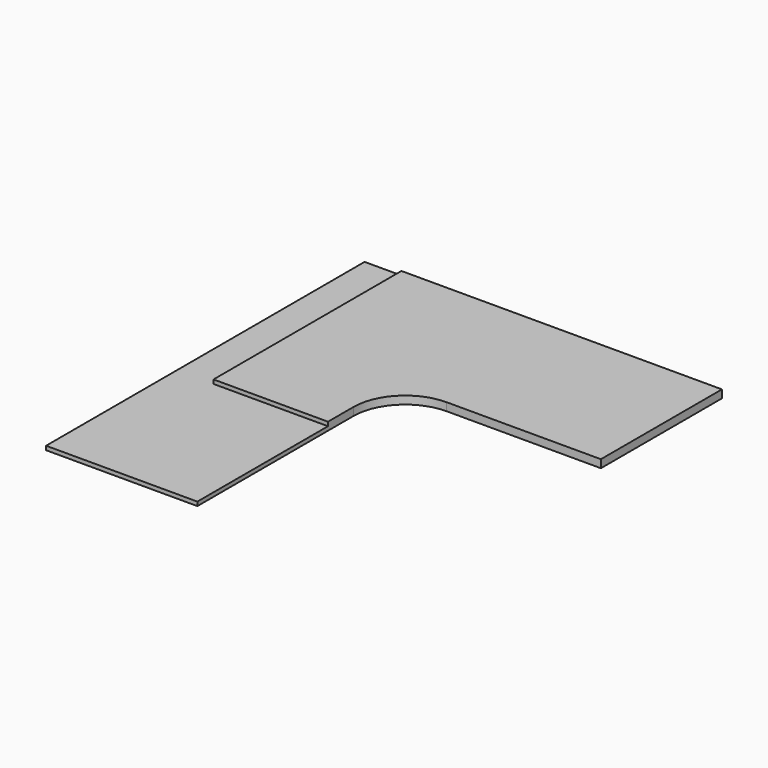
from build123d import *

# Parameters (mm, degrees)
F5_DEPTH = 20
F6_DEPTH = 20


# Not quite as in the source:
# - the program builds the solid bodies; features that only make, move or delete a surface that nothing else refers to are left out


with BuildPart() as f5:
    # F4 (on offset) → F5 (new body)
    with BuildSketch(Plane.XY.offset(720)):
        with BuildLine():
            ThreePointArc((0, -260), (76.1522368915, -76.1522368915), (260, 0))
            Line((260, 0), (1035, 0))
            Line((1035, 0), (1035, 760))
            Line((1035, 760), (-575, 760))
            Line((-575, 760), (-575, -420))
            Line((-575, -420), (0, -420))
            Line((0, -420), (0, -260))
        make_face()
    extrude(amount=F5_DEPTH)

    # F4 (on offset) → F6 (join)
    with BuildSketch(Plane.XY.offset(720)):
        with BuildLine():
            ThreePointArc((0, -260), (76.1522368915, -76.1522368915), (260, 0))
            Line((260, 0), (1035, 0))
            Line((1035, 0), (1035, 760))
            Line((1035, 760), (-575, 760))
            Line((-575, 760), (-575, -420))
            Line((-575, -420), (0, -420))
            Line((0, -420), (0, -260))
        make_face()
        Polygon((0, -1240), (0, -420), (-575, -420), (-575, 760), (-760, 760), (-760, -1240), align=None)
    extrude(amount=-F6_DEPTH)


solid = f5.part
